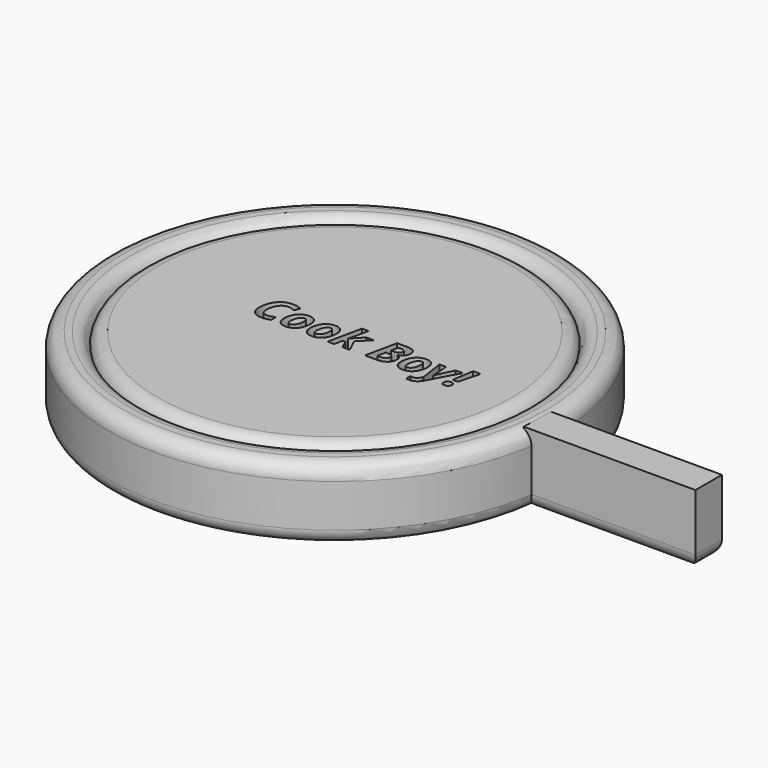
from build123d import *

# Parameters (mm, degrees)
F0_R          = 80.2417665351
F1_DEPTH      = 25.4
F2_R          = 67.8144377134
F3_DEPTH      = 25.4
F4_R          = 5.08
F5_R          = 67.991167514
F6_DEPTH      = 25.4
F8_R          = 68.2177223195
F9_DEPTH      = 12.7
F10_R         = 5.08
F11_TEXT_SIZE = 15.9001126627
F12_DEPTH     = 6.35
F14_DEPTH     = 25.4
F15_R         = 5.08


# Not quite as in the source:
# - a fillet or chamfer that OpenCascade refuses, or shapes differently, is made with other operations: its cross-section is extruded or revolved along the edge and cut away or added
# - a length typed as a fraction of an inch, garbled in the dataset ("3 / 203.2 mm" for 3/8 in), is restored
# - Text() gives the source's letters only with a copy of the font that has no kerning and outlines rounded to 1/6400 em; it was checked with that copy


with BuildPart() as f1:
    # F0 (on Top) → F1 (new body)
    with BuildSketch(Plane.XY):
        Circle(F0_R)
    extrude(amount=F1_DEPTH)

    # F2 (on face) → F3 (cut)
    with BuildSketch(Plane.XY.offset(25.4)):
        Circle(F2_R)
    extrude(amount=-F3_DEPTH, mode=Mode.SUBTRACT)

    # F4
    f4_edges = [f1.edges().sort_by_distance(p)[0] for p in [
        (-80.241767, 0, 25.4),
        (-67.814438, 0, 25.4),
    ]]
    fillet(f4_edges, radius=F4_R)

    # F5 (on Top) → F6 (join)
    with BuildSketch(Plane.XY):
        Circle(F5_R)
    extrude(amount=F6_DEPTH)

    # F7: fillet of radius 5.08 on 1 edges, made by hand

    # F7_s1 → F7_t2 (revolve, cut)
    with BuildSketch(Plane.XZ):
        with BuildLine():
            ThreePointArc((67.991167514, 21.6482851167), (66.174862783, 24.3544818994), (63.0878973145, 25.4))
            Line((63.0878973145, 25.4), (67.991167514, 25.4))
            Line((67.991167514, 25.4), (67.991167514, 21.6482851167))
        make_face()
    revolve(axis=Axis((0, 0, 25.4), (0, 0, 1)), mode=Mode.SUBTRACT)

    # F8 (on face) → F9 (cut)
    with BuildSketch(Plane(origin=(0, 0, 0), x_dir=(1, 0, 0), z_dir=(0, 0, -1))):
        Circle(F8_R)
    extrude(amount=-F9_DEPTH, mode=Mode.SUBTRACT)

    # F10
    f10_edges = [f1.edges().sort_by_distance(p)[0] for p in [
        (-80.241767, 0, 0),
        (-68.217722, 0, 0),
    ]]
    fillet(f10_edges, radius=F10_R)

    # F11 (on face) → F12 (cut)
    with BuildSketch(Plane.XY.offset(25.4)):
        with Locations((-26.5324302018, -5.8527537622)):
            Text('Cook Boy!', F11_TEXT_SIZE, font='Open Sans', font_style=FontStyle.BOLDITALIC, text_align=(TextAlign.LEFT, TextAlign.BOTTOM))
    extrude(amount=-F12_DEPTH, mode=Mode.SUBTRACT)


with BuildPart() as f14:
    # F13 (on Top) → F14 (new body)
    with BuildSketch(Plane.XY):
        Polygon((76.7222195864, 0), (76.5213742852, -11.7493458092), (137.577816844, -11.7493458092), (137.577816844, 0), align=None)
    extrude(amount=F14_DEPTH)

    # F15
    f15_edges = [f14.edges().sort_by_distance(p)[0] for p in [
        (76.621797, -5.874673, 0),
        (107.049596, -11.749346, 0),
        (137.577817, -5.874673, 0),
        (107.150018, 0, 0),
    ]]
    fillet(f15_edges, radius=F15_R)


solid = Compound([f1.part, f14.part])
